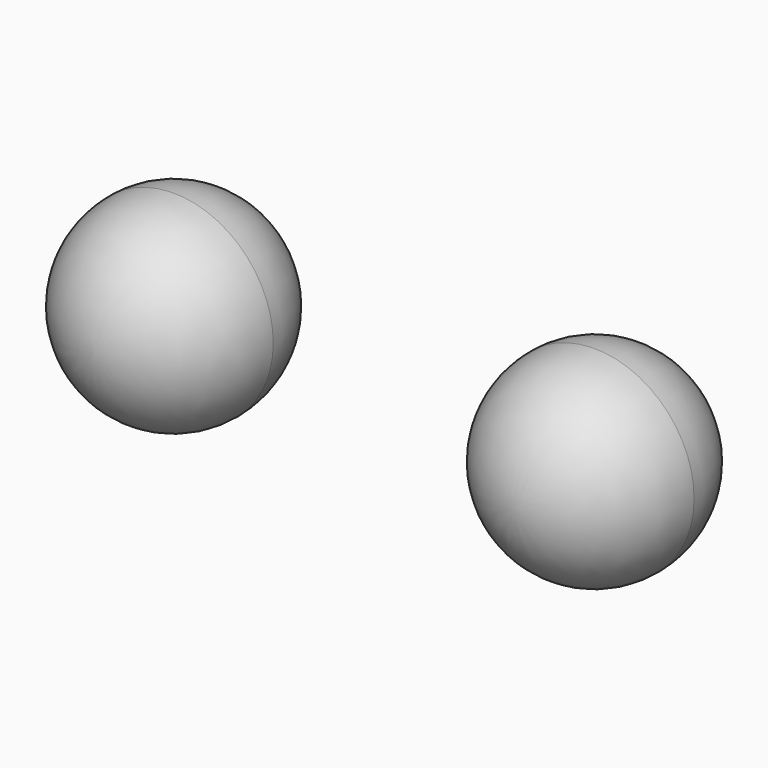
from build123d import *

# Parameters (mm, degrees)
F0_R     = 57.15
F1_DEPTH = 57.15
F2_R     = 57.14999
F2_2_R   = 57.14999


# Not quite as in the source:
# - a fillet or chamfer is up to 0.001 mm smaller than in the source, because OpenCascade refuses the exact size


with BuildPart() as f1:
    # F0 (on Front) → F1 (new body, symmetric)
    with BuildSketch(Plane.XZ):
        with Locations((120.65, 0)):
            Circle(F0_R)
    extrude(amount=F1_DEPTH, both=True)

    # F2 (radius 57.15 in the source; OpenCascade refuses exactly that, so slightly less here)
    f2_edges = [f1.edges().sort_by_distance(p)[0] for p in [
        (63.5, 57.15, 0),
        (63.5, -57.15, 0),
    ]]
    fillet(f2_edges, radius=F2_R)


with BuildPart() as f1b:
    # F0 (on Front) → F1, piece 2 (new body, symmetric)
    with BuildSketch(Plane.XZ):
        with Locations((-120.65, 0)):
            Circle(F0_R)
    extrude(amount=F1_DEPTH, both=True)

    # F2#2 (radius 57.15 in the source; OpenCascade refuses exactly that, so slightly less here)
    f2_2_edges = [f1b.edges().sort_by_distance(p)[0] for p in [
        (-177.8, -57.15, 0),
        (-177.8, 57.15, 0),
    ]]
    fillet(f2_2_edges, radius=F2_2_R)


solid = Compound([f1.part, f1b.part])
